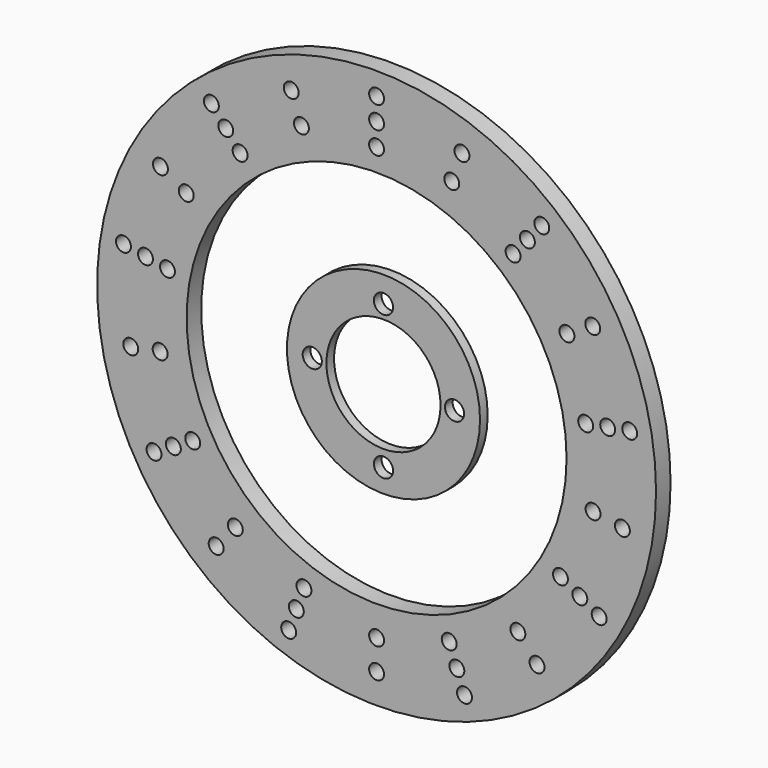
from build123d import *

# Parameters (mm, degrees)
F0_R            = 148.336
F0_R_2          = 100.838
F3_DEPTH        = 9.652
F2_R            = 3.9624
F4_DEPTH        = 9.653
F4_COPIES_COUNT = 9
F6_D            = 7.9248
F6_COPIES_COUNT = 9
F0_R_3          = 51.2445
F0_R_4          = 30.2895
F7_DEPTH        = 5.08
F8_D            = 10.16


# Not quite as in the source:
# - a pattern or mirror of a feature is missing from the dataset's text; its kind, count and spacing are read off the source's solid


with BuildPart() as f3:
    # F0 (on Front) → F3 (new body)
    with BuildSketch(Plane.XZ):
        Circle(F0_R)
        Circle(F0_R_2, mode=Mode.SUBTRACT)
    extrude(amount=F3_DEPTH)

    # F2 (on face) → F4 (cut, through all)
    with BuildSketch(Plane.XZ):
        with Locations((0, 112.6998)):
            Circle(F2_R)
        with Locations((0, 124.5616)):
            Circle(F2_R)
        with Locations((0, 136.4234)):
            Circle(F2_R)
    f4 = extrude(amount=F4_DEPTH, mode=Mode.SUBTRACT)

    # F4_copies: F4 ×9 about axis
    f4_copies_axis = Axis((0, 0, 0), (0, 1, 0))
    for i in range(1, F4_COPIES_COUNT):
        add(f4.rotate(f4_copies_axis, i * 360 / F4_COPIES_COUNT), mode=Mode.SUBTRACT)

    # F6 (through all)
    with Locations(Plane(origin=(0, 0, 0), x_dir=(1, 0, 0), z_dir=(0, 1, 0))):
        with Locations((0, 116.6622), (0, 132.4864)):
            f6 = Hole(F6_D / 2)

    # F6_copies: F6 ×9 about axis
    f6_copies_axis = Axis((0, 0, 0), (0, 1, 0))
    for i in range(1, F6_COPIES_COUNT):
        add(f6.rotate(f6_copies_axis, i * 360 / F6_COPIES_COUNT), mode=Mode.SUBTRACT)


with BuildPart() as f7:
    # F0 (on Front) → F7 (new body)
    with BuildSketch(Plane.XZ):
        Circle(F0_R_3)
        Circle(F0_R_4, mode=Mode.SUBTRACT)
    extrude(amount=F7_DEPTH)

    # F8 (through all)
    with Locations(Plane(origin=(0, 0, 0), x_dir=(1, 0, 0), z_dir=(0, 1, 0))):
        with Locations((0, -37.5412), (37.7119863628, 0), (0, 38.8407654956), (-37.8069085799, 0)):
            Hole(F8_D / 2)


solid = Compound([f3.part, f7.part])
